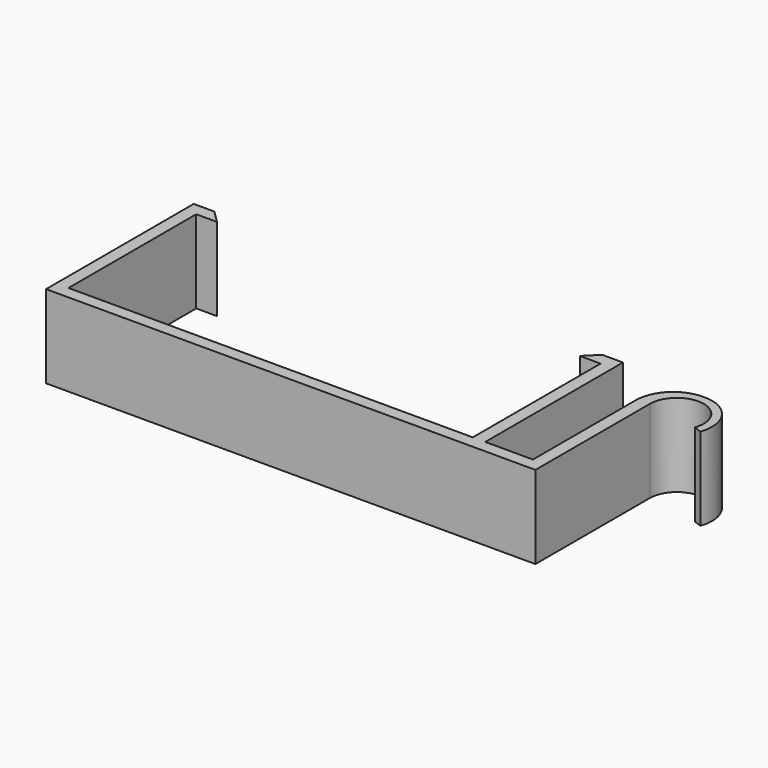
from build123d import *

# Parameters (mm, degrees)
F1_DEPTH = 20
F2_SIZE  = 2.99999
F3_R     = 9


# Not quite as in the source:
# - a fillet or chamfer is up to 0.001 mm smaller than in the source, because OpenCascade refuses the exact size


with BuildPart() as f1:
    # F0 (on Top) → F1 (new body)
    with BuildSketch(Plane.XY):
        with BuildLine():
            Line((0, 40), (0, 0))
            Line((0, 0), (-11.5, 0))
            Line((-11.5, 0), (-11.5, 41.5))
            Line((-11.5, 41.5), (-19.5, 41.5))
            Line((-19.5, 41.5), (-19.5, 38.5))
            Line((-19.5, 38.5), (-14.5, 38.5))
            Line((-14.5, 38.5), (-14.5, 0))
            Line((-14.5, 0), (-112, 0))
            Line((-112, 0), (-112, 38.5))
            Line((-112, 38.5), (-107, 38.5))
            Line((-107, 38.5), (-107, 41.5))
            Line((-107, 41.5), (-115, 41.5))
            Line((-115, 41.5), (-115, -3))
            Line((-115, -3), (3, -3))
            Line((3, -3), (3, 31.5))
            ThreePointArc((3, 31.5), (10.6287131548, 37.9012503946), (15.6080020351, 29.2768690684))
            Line((15.6080020351, 29.2768690684), (17.4873872767, 28.5928287817))
            ThreePointArc((17.4873872767, 28.5928287817), (16.4627923765, 36.375399709), (9.5, 40))
            Line((9.5, 40), (3, 40))
            Line((3, 40), (0, 40))
        make_face()
    extrude(amount=F1_DEPTH)

    # F2 (size 3 in the source; OpenCascade refuses exactly that, so slightly less here)
    f2_edges = [f1.edges().sort_by_distance(p)[0] for p in [
        (-107, 41.5, 10),
        (-19.5, 41.5, 10),
    ]]
    chamfer(f2_edges, length=F2_SIZE)

    # F3
    f3_edges = [f1.edges().sort_by_distance(p)[0] for p in [
        (0, 40, 10),
    ]]
    fillet(f3_edges, radius=F3_R)


solid = f1.part
